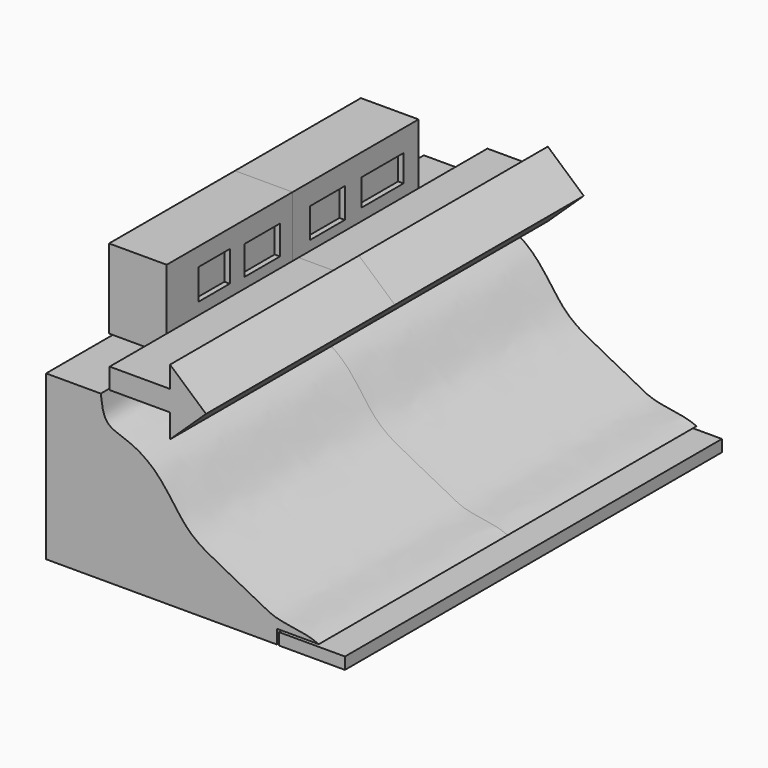
from build123d import *

# Parameters (mm, degrees)
F0_W     = 21.2485753
F0_H     = 152.0810052752
F1_DEPTH = 3.81
F3_DEPTH = 76.2
F2_W     = 19.4977223873
F2_H     = 6.6637769341
F4_DEPTH = 76.2
F5_W     = 18.6125934124
F5_H     = 25.6022065878
F6_DEPTH = 50.8
F7_DEPTH = 50.8
F8_W     = 14.3147837371
F8_H     = 9.378656745
F8_W_2   = 14.0679730102
F8_H_2   = 9.6254572272
F8_W_3   = 12.587139383
F8_H_3   = 9.8722651601
F8_W_4   = 17.029652372
F8_H_4   = 8.6382329464
F9_DEPTH = 58.42


with BuildPart() as f1:
    # F0 (on Top) → F1 (new body)
    with BuildSketch(Plane.XY):
        with Locations((10.62428765, -0.267278403)):
            Rectangle(F0_W, F0_H)
    extrude(amount=F1_DEPTH)


with BuildPart() as f3:
    # F2 (on Front) → F3 (new body)
    with BuildSketch(Plane.XZ):
        with BuildLine():
            Line((-57.6507113874, 52.8162680566), (-75.2964168787, 52.8162680566))
            Line((-75.2964168787, 52.8162680566), (-75.2964168787, 0))
            Line((-75.2964168787, 0), (-0.846029463, 0))
            Line((-0.846029463, 0), (-0.846029463, 4.4855900342))
            Line((-0.846029463, 4.4855900342), (0, 4.4855900342))
            Line((0, 4.4855900342), (12.7145235892, 4.4855900342))
            add(Edge.make_bspline(
                [(-57.6507113874, 52.8162680566), (-57.3076574479, 49.9294208495), (-56.6267364551, 44.1968150065), (-48.3342084307, 42.576740226), (-38.0818843322, 36.1305714757), (-30.3544979342, 22.4931937459), (-19.7634057619, 16.912441387), (-6.7248199885, 10.2621660981), (-0.3365370443, 6.6140396), (8.4946691957, 6.3613474044), (12.7145235892, 4.4855900342)],
                knots=[0, 0, 0, 0, 0.1056642831, 0.2074992162, 0.338577851, 0.4857937218, 0.6179620961, 0.7603575547, 0.8635138744, 1, 1, 1, 1], degree=3))
        make_face()
    extrude(amount=F3_DEPTH)


with BuildPart() as f3b:
    # F2 (on Front) → F3, piece 2 (new body)
    with BuildSketch(Plane.XZ):
        with Locations((-45.0337249786, 58.0747127533)):
            Rectangle(F2_W, F2_H)
        Polygon((-35.2848637849, 68.3171860874), (-35.2848637849, 61.4066012204), (-35.2848637849, 54.7428242862), (-35.2848637849, 47.091819346), (-23.6849524081, 58.0747127533), align=None)
    extrude(amount=F3_DEPTH)


with BuildPart() as f4:
    # F4 (new): a face of the model
    f4_faces = [f3.part.faces().sort_by_distance(p)[0] for p in [
        (-48.0221712307, 0, 19.9820449464),
    ]]
    extrude(f4_faces, amount=F4_DEPTH)


with BuildPart() as f4b:
    # F4#2 (new): a face of the model
    f4_2_faces = [f3b.part.faces().sort_by_distance(p)[0] for p in [
        (-38.4095254278, 0, 57.954636592),
    ]]
    extrude(f4_2_faces, amount=F4_DEPTH)


with BuildPart() as f6:
    # F5 (on Front) → F6 (new body)
    with BuildSketch(Plane.XZ):
        with Locations((-65.9901201725, 66.6045919061)):
            Rectangle(F5_W, F5_H)
    extrude(amount=F6_DEPTH)


with BuildPart() as f7:
    # F7 (new): a face of the model
    f7_faces = [f6.part.faces().sort_by_distance(p)[0] for p in [
        (-65.9901201725, 0, 66.6045919061),
    ]]
    extrude(f7_faces, amount=F7_DEPTH)


with BuildPart() as f9_tool:
    # F8 (on Right) → F9 (new body)
    with BuildSketch(Plane.YZ):
        with Locations((-12.2708184645, 67.8704231977)):
            Rectangle(F8_W, F8_H)
        with Locations((14.0140862204, 67.7470229566)):
            Rectangle(F8_W_2, F8_H_2)
        with Locations((-31.6451368853, 68.610843271)):
            Rectangle(F8_W_3, F8_H_3)
        with Locations((36.2266814336, 67.9938271642)):
            Rectangle(F8_W_4, F8_H_4)
    extrude(amount=-F9_DEPTH)


with BuildPart() as f6_1:
    add(f6.part)

    # F9: cut by f9_tool
    add(f9_tool.part, mode=Mode.SUBTRACT)


with BuildPart() as f7_1:
    add(f7.part)

    # F9: cut by f9_tool
    add(f9_tool.part, mode=Mode.SUBTRACT)


solid = Compound([f1.part, f3.part, f3b.part, f4.part, f4b.part, f6_1.part, f7_1.part])
